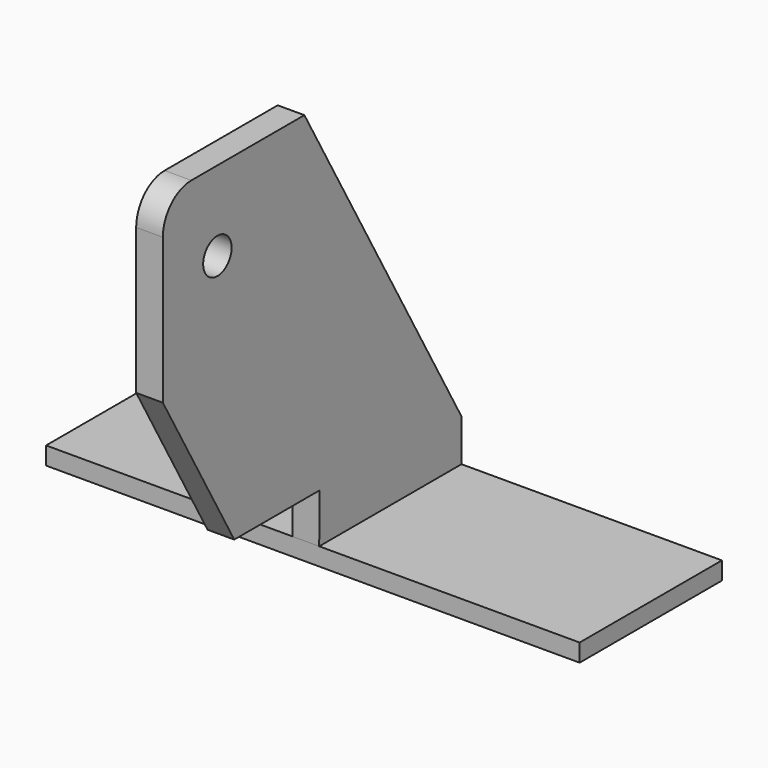
from build123d import *

# Parameters (mm, degrees)
F0_W     = 30
F0_H     = 10
F1_DEPTH = 1
F2_R     = 1
F3_DEPTH = 0.75


# Not quite as in the source:
# - a feature of the source that left no trace in its solid (it failed there, or was rolled back) is left out


with BuildPart() as f1:
    # F0 (on Top) → F1 (new body)
    with BuildSketch(Plane.XY):
        with Locations((0.392307792, 0)):
            Rectangle(F0_W, F0_H)
    extrude(amount=F1_DEPTH)

    # F2 (on Right) → F3 (join, symmetric)
    with BuildSketch(Plane.YZ):
        with BuildLine():
            Line((-5, 1), (5, 1))
            Line((5, 1), (5, 3.3628055826))
            Line((5, 3.3628055826), (-6.0430504382, 22.7664429694))
            Line((-6.0430504382, 22.7664429694), (-13.9894526005, 22.7664429694))
            ThreePointArc((-13.9894526005, 22.7664429694), (-15.4036661629, 22.1806565318), (-15.9894526005, 20.7664429694))
            Line((-15.9894526005, 20.7664429694), (-15.9894526005, 12.5754568726))
            Line((-15.9894526005, 12.5754568726), (-10.9724997157, 3.7602173598))
            Line((-10.9724997157, 3.7602173598), (-4.9831885844, 3.7602173598))
            Line((-4.9831885844, 3.7602173598), (-5, 1))
        make_face()
        with Locations((-12.1576432139, 18.2824078947)):
            Circle(F2_R, mode=Mode.SUBTRACT)
    extrude(amount=F3_DEPTH, both=True)


solid = f1.part
